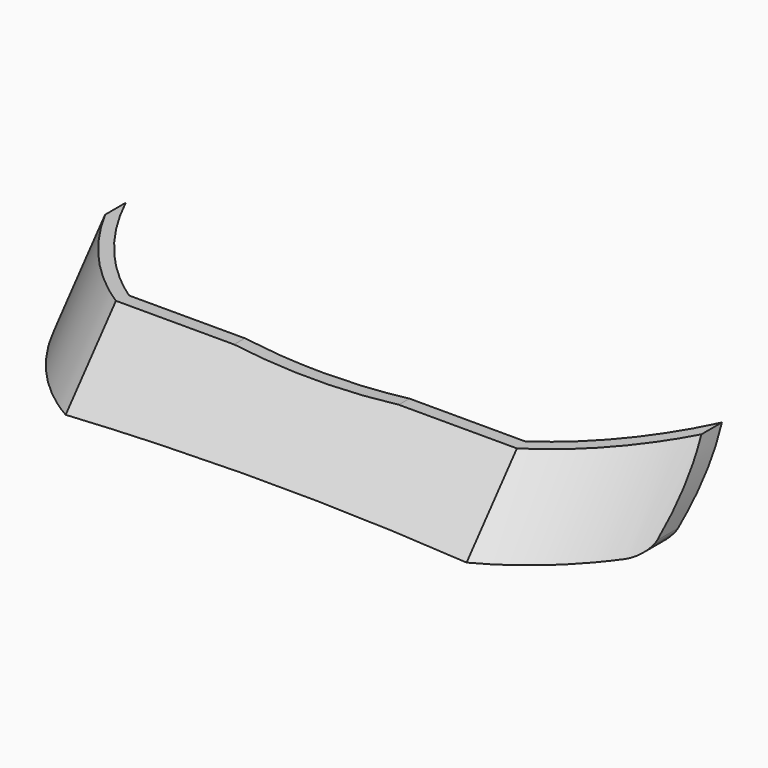
from build123d import *

# Parameters (mm, degrees)
F1_DEPTH      = 40
F1_DEPTH_BACK = 11
F4_DEPTH      = 35
F4_DEPTH_BACK = 27.9057510197
F5_T1_DEPTH   = 14.6143927182
F5_T3_DEPTH   = 14.6250082056


# Not quite as in the source:
# - a fillet or chamfer that OpenCascade refuses, or shapes differently, is made with other operations: its cross-section is extruded or revolved along the edge and cut away or added


with BuildPart() as f1:
    # F0 (on Front) → F1 (new body, two sides)
    with BuildSketch(Plane.XZ) as f1_sk:
        with BuildLine():
            Line((-16, 15.5), (-58, 15.5))
            ThreePointArc((-58, 15.5), (-58.5026261084, 7.75), (-58, 0))
            ThreePointArc((-58, 0), (-0.000843128, 1.7124660629), (58, 0.0580978101))
            ThreePointArc((58, 0.0580978101), (58.5026261084, 7.8080978101), (58, 15.5580978101))
            Line((58, 15.5580978101), (16, 15.5580978101))
            ThreePointArc((16, 15.5580978101), (0.0011638232, 14.8880205552), (-16, 15.5))
        make_face()
    extrude(amount=F1_DEPTH)
    extrude(f1_sk.sketch, amount=-F1_DEPTH_BACK)

    # F3 (on face) → F4 (cut, two sides)
    with BuildSketch(Plane(origin=(0, -8.8661687739, -10.5662884888), x_dir=(1, 0, 0), z_dir=(0, -0.6427876097, -0.7660444431))) as f4_sk:
        with BuildLine():
            Line((38.4965417924, 21), (0, 20.9813332936))
            Line((0, 20.9813332936), (-38.534011751, 20.9813332936))
            ThreePointArc((-38.534011751, 20.9813332936), (-51.7445439017, 11.0585633209), (-61, -2.6277822851))
            Line((-61, -2.6277822851), (-61, -10.626510717))
            Line((-61, -10.626510717), (-61, -28.2158330083))
            Line((-61, -28.2158330083), (0, -28.2158330083))
            Line((0, -28.2158330083), (61, -28.2158330083))
            Line((61, -28.2158330083), (61, -12.4673116952))
            Line((61, -12.4673116952), (61, -2.6264255467))
            ThreePointArc((61, -2.6264255467), (51.7297238243, 11.0740614176), (38.4965417924, 21))
        make_face()
        with BuildLine():
            Line((61, 1.9813332936), (61, 22.9813332936))
            Line((61, 22.9813332936), (61, 52.9813332936))
            Line((61, 52.9813332936), (-61, 52.9813332936))
            Line((-61, 52.9813332936), (-61, 22.9813332936))
            Line((-61, 22.9813332936), (-61, 1.9813332936))
            ThreePointArc((-61, 1.9813332936), (-51.6354627813, 14.1946752549), (-39, 22.9813332936))
            Line((-39, 22.9813332936), (39, 22.9813332936))
            ThreePointArc((39, 22.9813332936), (51.6354627813, 14.1946752549), (61, 1.9813332936))
        make_face()
    extrude(amount=-F4_DEPTH, mode=Mode.SUBTRACT)
    extrude(f4_sk.sketch, amount=F4_DEPTH_BACK, mode=Mode.SUBTRACT)

    # F5: fillet of radius 2 on 2 edges, made by hand

    # F5_s2 → F5_t1 (cut)
    with BuildSketch(Plane.XZ.offset(-0.9773730981)):
        with BuildLine():
            ThreePointArc((56.1159001591, 0.164829526), (57.5290135561, 0.6434770054), (58.2176321612, 1.9670318018))
            ThreePointArc((58.2176321612, 1.9670318018), (58.1164574753, 1.0116936322), (58, 0.0580978101))
            ThreePointArc((58, 0.0580978101), (57.0579752565, 0.1119081086), (56.1159001591, 0.164829526))
        make_face()
    extrude(amount=F5_T1_DEPTH, mode=Mode.SUBTRACT)

    # F5_s4 → F5_t3 (cut)
    with BuildSketch(Plane.XZ.offset(-0.9343439765)):
        with BuildLine():
            ThreePointArc((-58.2178227579, 1.9108828482), (-57.5284634735, 0.5866337247), (-56.1140880268, 0.1087278139))
            ThreePointArc((-56.1140880268, 0.1087278139), (-57.0570696874, 0.0548092283), (-58, 0))
            ThreePointArc((-58, 0), (-58.1165683708, 0.9545685987), (-58.2178227579, 1.9108828482))
        make_face()
    extrude(amount=F5_T3_DEPTH, mode=Mode.SUBTRACT)


solid = f1.part
